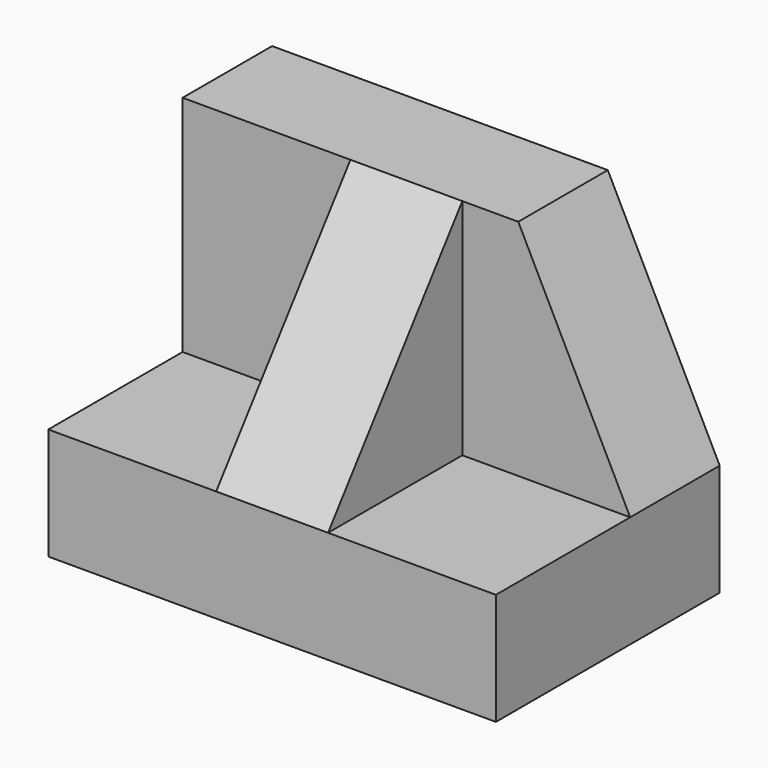
from build123d import *

# Parameters (mm, degrees)
F0_W     = 50.8
F0_H     = 38.1
F1_DEPTH = 31.75
F3_DEPTH = 12.7
F4_W     = 19.05
F4_H     = 25.4
F5_DEPTH = 19.05
F7_DEPTH = 12.7
F8_W     = 19.05
F8_H     = 25.4
F9_DEPTH = 19.05


with BuildPart() as f1:
    # F0 (on Front) → F1 (new body)
    with BuildSketch(Plane.XZ):
        with Locations((-32.8861247392, 25.7318585645)):
            Rectangle(F0_W, F0_H)
    extrude(amount=F1_DEPTH)

    # F2 (on face) → F3 (cut)
    with BuildSketch(Plane(origin=(0, 0, 0), x_dir=(-1, 0, 0), z_dir=(0, 1, 0))):
        Polygon((7.4861247392, 19.3818585645), (20.1861247392, 44.7818585645), (7.4861247392, 44.7818585645), align=None)
    extrude(amount=-F3_DEPTH, mode=Mode.SUBTRACT)

    # F4 (on face) → F5 (cut)
    with BuildSketch(Plane.YZ.offset(-7.4861247392)):
        with Locations((-22.225, 32.0818585645)):
            Rectangle(F4_W, F4_H)
    extrude(amount=-F5_DEPTH, mode=Mode.SUBTRACT)

    # F6 (on face) → F7 (cut)
    with BuildSketch(Plane.YZ.offset(-26.5361247392)):
        Polygon((-31.75, 19.3818585645), (-12.7, 44.7818585645), (-31.75, 44.7818585645), align=None)
    extrude(amount=-F7_DEPTH, mode=Mode.SUBTRACT)

    # F8 (on face) → F9 (cut)
    with BuildSketch(Plane.XZ.offset(31.75)):
        with Locations((-48.7611247392, 32.0818585645)):
            Rectangle(F8_W, F8_H)
    extrude(amount=-F9_DEPTH, mode=Mode.SUBTRACT)


solid = f1.part
